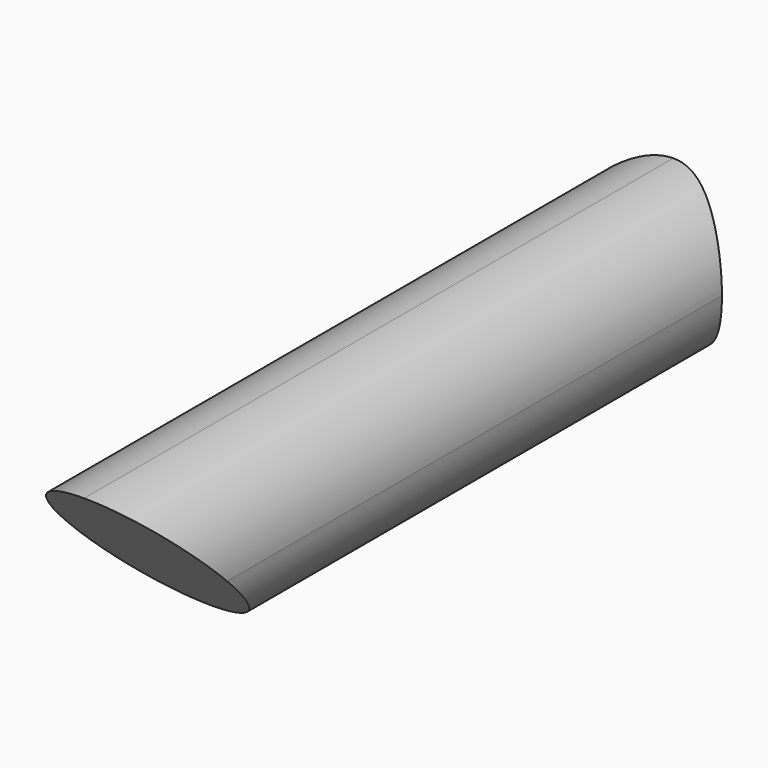
from build123d import *

# Parameters (mm, degrees)
F0_W     = 33
F0_H     = 33
F1_DEPTH = 166
F3_DEPTH = 100
F4_R     = 16.49999
F6_DEPTH = 50


# Not quite as in the source:
# - a fillet or chamfer is up to 0.001 mm smaller than in the source, because OpenCascade refuses the exact size


with BuildPart() as f1:
    # F0 (on Front) → F1 (new body)
    with BuildSketch(Plane.XZ):
        Rectangle(F0_W, F0_H)
    extrude(amount=F1_DEPTH)

    # F2 (on face) → F3 (cut)
    with BuildSketch(Plane.YZ.offset(16.5)):
        Polygon((-133, -16.5), (-166, 16.5), (-166, -16.5), align=None)
    extrude(amount=-F3_DEPTH, mode=Mode.SUBTRACT)

    # F4 (radius 16.5 in the source; OpenCascade refuses exactly that, so slightly less here)
    f4_edges = [f1.edges().sort_by_distance(p)[0] for p in [
        (-16.5, -83, 16.5),
        (-16.5, -66.5, -16.5),
        (16.5, -83, 16.5),
        (16.5, -66.5, -16.5),
    ]]
    fillet(f4_edges, radius=F4_R)

    # F5 (on Right) → F6 (cut, symmetric)
    with BuildSketch(Plane.YZ):
        with BuildLine():
            Line((0, -21), (0, 0))
            Line((0, 0), (0, 21))
            ThreePointArc((0, 21), (-21, 0), (0, -21))
        make_face()
    extrude(amount=F6_DEPTH, both=True, mode=Mode.SUBTRACT)


solid = f1.part
